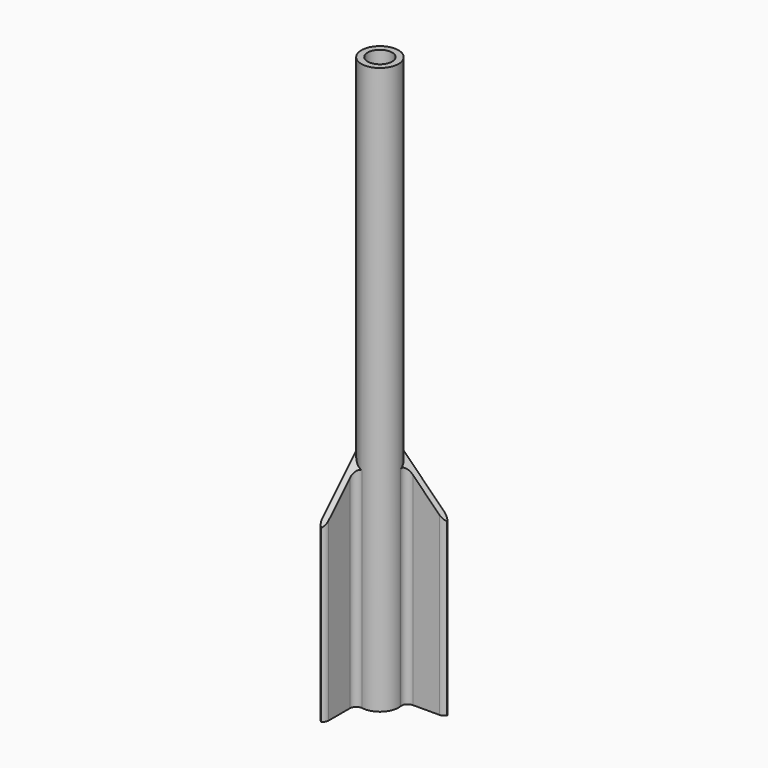
from build123d import *

# Parameters (mm, degrees)
F0_R         = 2.95
F1_DEPTH     = 95
F3_DEPTH     = 35
F4_T4_DEPTH  = 1
F4_S5_R      = 2.95
F4_T6_DEPTH  = 8
F4_T10_DEPTH = 1
F4_S11_R     = 2.95
F4_T12_DEPTH = 8
F5_T4_DEPTH  = 37.2779404698
F5_T9_DEPTH  = 35.3377138687
F5_T14_DEPTH = 35.3377138687
F5_T19_DEPTH = 37.2779404698
F5_T21_DEPTH = 32
F9_R         = 1
F10_DEPTH    = 12.5
F11_DEPTH    = 5
F12_R        = 1.95
F13_DEPTH    = 20
F15_D        = 1.8
F15_DEPTH    = 5
F15_TIP      = 0.5407745571


# Not quite as in the source:
# - a fillet or chamfer that OpenCascade refuses, or shapes differently, is made with other operations: its cross-section is extruded or revolved along the edge and cut away or added


with BuildPart() as f1:
    # F0 (on Top) → F1 (new body)
    with BuildSketch(Plane.XY):
        Circle(F0_R)
    extrude(amount=F1_DEPTH)

    # F2 (on Top) → F3 (join)
    with BuildSketch(Plane.XY):
        Polygon((1.3030903237, 2.6465932079), (2.4476990844, 1.6465932079), (9.1030903237, 1.6465932079), (9.1030903237, 2.6465932079), align=None)
        Polygon((-2.6465932079, -9.1030903237), (-1.6465932079, -9.1030903237), (-1.6465932079, -2.4476990844), (-2.6465932079, -1.3030903237), align=None)
    extrude(amount=F3_DEPTH)

    # F4: chamfer of 8 on 2 edges, made by hand


with BuildPart() as f4_tool2:
    # F4_s3 → F4_t4 (new body)
    with BuildSketch(Plane.XZ.offset(-1.6465932079)):
        with BuildLine():
            Line((0.8768161537, 35.22627417), (9.3293644937, 26.77372583))
            Line((9.3293644937, 26.77372583), (9.4893644937, 26.77372583))
            ThreePointArc((9.4893644937, 26.77372583), (9.2630903237, 30.886862915), (9.2630903237, 35))
            Line((9.2630903237, 35), (9.1030903237, 35.16))
            ThreePointArc((9.1030903237, 35.16), (4.9899532387, 35.16), (0.8768161537, 35.38627417))
            Line((0.8768161537, 35.38627417), (0.8768161537, 35.22627417))
        make_face()
    extrude(amount=-F4_T4_DEPTH)

    # F4_s5 → F4_t6 (cut, symmetric)
    with BuildSketch(Plane.XY.offset(31.1)):
        Circle(F4_S5_R)
    extrude(amount=F4_T6_DEPTH, both=True, mode=Mode.SUBTRACT)


with BuildPart() as f1_1:
    add(f1.part)

    # F4_t1: cut F4_tool2
    add(f4_tool2.part, mode=Mode.SUBTRACT)


with BuildPart() as f4_tool8:
    # F4_s9 → F4_t10 (new body)
    with BuildSketch(Plane.YZ.offset(-2.6465932079)):
        with BuildLine():
            Line((-0.8768161537, 35.22627417), (-9.3293644937, 26.77372583))
            Line((-9.3293644937, 26.77372583), (-9.4893644937, 26.77372583))
            ThreePointArc((-9.4893644937, 26.77372583), (-9.2630903237, 30.886862915), (-9.2630903237, 35))
            Line((-9.2630903237, 35), (-9.1030903237, 35.16))
            ThreePointArc((-9.1030903237, 35.16), (-4.9899532387, 35.16), (-0.8768161537, 35.38627417))
            Line((-0.8768161537, 35.38627417), (-0.8768161537, 35.22627417))
        make_face()
    extrude(amount=F4_T10_DEPTH)

    # F4_s11 → F4_t12 (cut, symmetric)
    with BuildSketch(Plane.XY.offset(31.1)):
        Circle(F4_S11_R)
    extrude(amount=F4_T12_DEPTH, both=True, mode=Mode.SUBTRACT)


with BuildPart() as f1_2:
    add(f1_1.part)

    # F4_t7: cut F4_tool8
    add(f4_tool8.part, mode=Mode.SUBTRACT)

    # F5: fillet of radius 1 on 8 edges, made by hand


with BuildPart() as f5_tool2:
    # F5_s3 → F5_t4 (new body)
    with BuildSketch(Plane.XY):
        with BuildLine():
            ThreePointArc((-0.4828987249, -2.9102076939), (-1.2932405295, -3.1339296566), (-1.6465932079, -3.8967187765))
            Line((-1.6465932079, -3.8967187765), (-1.6465932079, -2.4476990844))
            ThreePointArc((-1.6465932079, -2.4476990844), (-1.0895698814, -2.7414115841), (-0.4828987249, -2.9102076939))
        make_face()
    extrude(amount=F5_T4_DEPTH)

    split(bisect_by=Plane(origin=(0, -18.0515451619, 18.0515451618), x_dir=(1, 0, 0), z_dir=(0, 0.7071067812, -0.7071067812)), keep=Keep.TOP)


with BuildPart() as f1_3:
    add(f1_2.part)

    # F5_t1: union F5_tool2
    add(f5_tool2.part)


with BuildPart() as f5_tool7:
    # F5_s8 → F5_t9 (new body)
    with BuildSketch(Plane.XY):
        with BuildLine():
            ThreePointArc((-2.723405054, -1.1338275494), (-2.6659841743, -1.3222015794), (-2.6465932079, -1.5181758712))
            Line((-2.6465932079, -1.5181758712), (-2.6465932079, -1.3030903237))
            ThreePointArc((-2.6465932079, -1.3030903237), (-2.6863325939, -1.2190640651), (-2.723405054, -1.1338275494))
        make_face()
    extrude(amount=F5_T9_DEPTH)

    split(bisect_by=Plane(origin=(0, -18.0515451619, 18.0515451618), x_dir=(1, 0, 0), z_dir=(0, 0.7071067812, -0.7071067812)), keep=Keep.TOP)


with BuildPart() as f1_4:
    add(f1_3.part)

    # F5_t6: union F5_tool7
    add(f5_tool7.part)


with BuildPart() as f5_tool12:
    # F5_s13 → F5_t14 (new body)
    with BuildSketch(Plane.XY):
        with BuildLine():
            ThreePointArc((1.1338275494, 2.723405054), (1.3222015794, 2.6659841743), (1.5181758712, 2.6465932079))
            Line((1.5181758712, 2.6465932079), (1.3030903237, 2.6465932079))
            ThreePointArc((1.3030903237, 2.6465932079), (1.2190640651, 2.6863325939), (1.1338275494, 2.723405054))
        make_face()
    extrude(amount=F5_T14_DEPTH)

    split(bisect_by=Plane(origin=(18.0515451619, 0, 18.0515451618), x_dir=(0, 1, 0), z_dir=(-0.7071067812, 0, -0.7071067812)), keep=Keep.TOP)


with BuildPart() as f1_5:
    add(f1_4.part)

    # F5_t11: union F5_tool12
    add(f5_tool12.part)


with BuildPart() as f5_tool17:
    # F5_s18 → F5_t19 (new body)
    with BuildSketch(Plane.XY):
        with BuildLine():
            ThreePointArc((2.9102076939, 0.4828987249), (3.1339296566, 1.2932405295), (3.8967187765, 1.6465932079))
            Line((3.8967187765, 1.6465932079), (2.4476990844, 1.6465932079))
            ThreePointArc((2.4476990844, 1.6465932079), (2.7414115841, 1.0895698814), (2.9102076939, 0.4828987249))
        make_face()
    extrude(amount=F5_T19_DEPTH)

    split(bisect_by=Plane(origin=(18.0515451619, 0, 18.0515451618), x_dir=(0, 1, 0), z_dir=(-0.7071067812, 0, -0.7071067812)), keep=Keep.TOP)


with BuildPart() as f1_6:
    add(f1_5.part)

    # F5_t16: union F5_tool17
    add(f5_tool17.part)

    # F5_s22 → F5_t21 (cut)
    with BuildSketch(Plane.XY.offset(-2.5)):
        with BuildLine():
            ThreePointArc((8.1030903237, 1.6465932079), (8.8101971049, 1.9394864268), (9.1030903237, 2.6465932079))
            Line((9.1030903237, 2.6465932079), (9.1030903237, 1.6465932079))
            Line((9.1030903237, 1.6465932079), (8.1030903237, 1.6465932079))
        make_face()
        with BuildLine():
            ThreePointArc((9.1030903237, 1.6465932079), (8.8101971049, 2.3536999891), (8.1030903237, 2.6465932079))
            Line((8.1030903237, 2.6465932079), (9.1030903237, 2.6465932079))
            Line((9.1030903237, 2.6465932079), (9.1030903237, 1.6465932079))
        make_face()
        with BuildLine():
            ThreePointArc((-2.6465932079, -8.1030903237), (-2.3536999891, -8.8101971049), (-1.6465932079, -9.1030903237))
            Line((-1.6465932079, -9.1030903237), (-2.6465932079, -9.1030903237))
            Line((-2.6465932079, -9.1030903237), (-2.6465932079, -8.1030903237))
        make_face()
        with BuildLine():
            ThreePointArc((-2.6465932079, -9.1030903237), (-1.9394864268, -8.8101971049), (-1.6465932079, -8.1030903237))
            Line((-1.6465932079, -8.1030903237), (-1.6465932079, -9.1030903237))
            Line((-1.6465932079, -9.1030903237), (-2.6465932079, -9.1030903237))
        make_face()
    extrude(amount=F5_T21_DEPTH, mode=Mode.SUBTRACT)

    # F9 (on 3pt) → F10 (cut, symmetric)
    with BuildSketch(Plane(origin=(0, 0, 0), x_dir=(0.7071067812, -0.7071067812, 0), z_dir=(-0.7071067812, -0.7071067812, 0))):
        Circle(F9_R)
    extrude(amount=F10_DEPTH, both=True, mode=Mode.SUBTRACT)

    # F11 (cut): a face of the model
    f11_faces = [f1_6.faces().sort_by_distance(p)[0] for p in [
        (0, 0, 95),
    ]]
    extrude(f11_faces, amount=-F11_DEPTH, mode=Mode.SUBTRACT)

    # F12 (on face) → F13 (cut)
    with BuildSketch(Plane.XY.offset(90)):
        Circle(F12_R)
    extrude(amount=-F13_DEPTH, mode=Mode.SUBTRACT)

    # F15
    with Locations(Plane.XY.offset(70)):
        with Locations((0, 0)):
            Hole(F15_D / 2, depth=F15_DEPTH)
            with Locations((0, 0, -(F15_DEPTH + F15_TIP / 2))):  # 118° drill point
                Cone(0, F15_D / 2, F15_TIP, mode=Mode.SUBTRACT)


solid = f1_6.part
